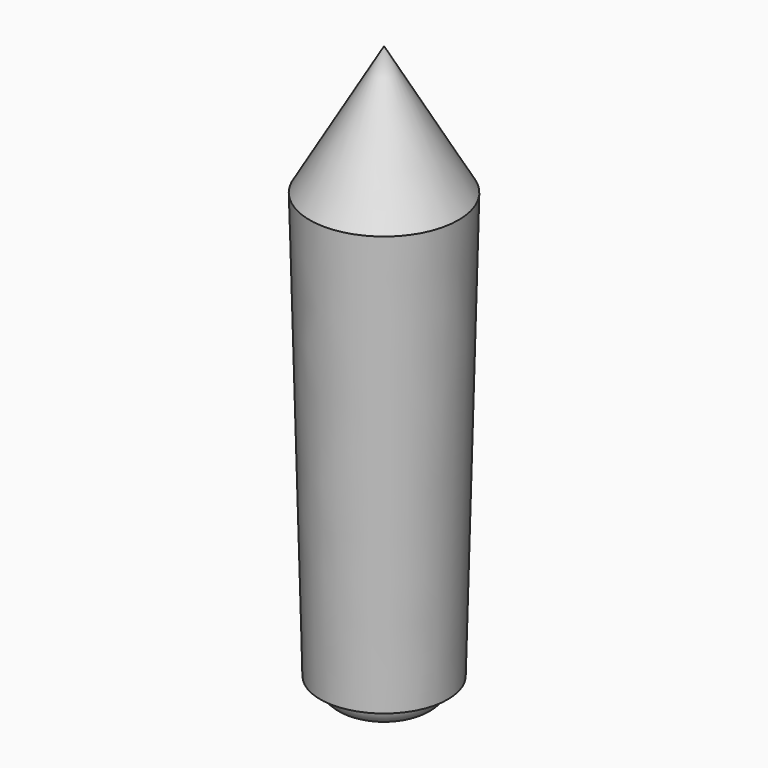
from build123d import *

# Parameters (mm, degrees)
F2_R = 3.99999


# Not quite as in the source:
# - a fillet or chamfer is up to 0.001 mm smaller than in the source, because OpenCascade refuses the exact size


with BuildPart() as f1:
    # F0 (on Front) → F1 (revolve)
    with BuildSketch(Plane.XZ):
        Polygon((14, 60.8242780692), (0, 85.0729893751), (0, -23.1757219308), (10, -23.1757219308), (10, -19.1757219308), (12, -19.1757219308), align=None)
    revolve(axis=Axis((0, 0, 30.9486337222), (0, 0, -1)))

    # F2 (radius 4 in the source; OpenCascade refuses exactly that, so slightly less here)
    f2_edges = [f1.edges().sort_by_distance(p)[0] for p in [
        (-10, 0, -23.175722),
    ]]
    fillet(f2_edges, radius=F2_R)


solid = f1.part
